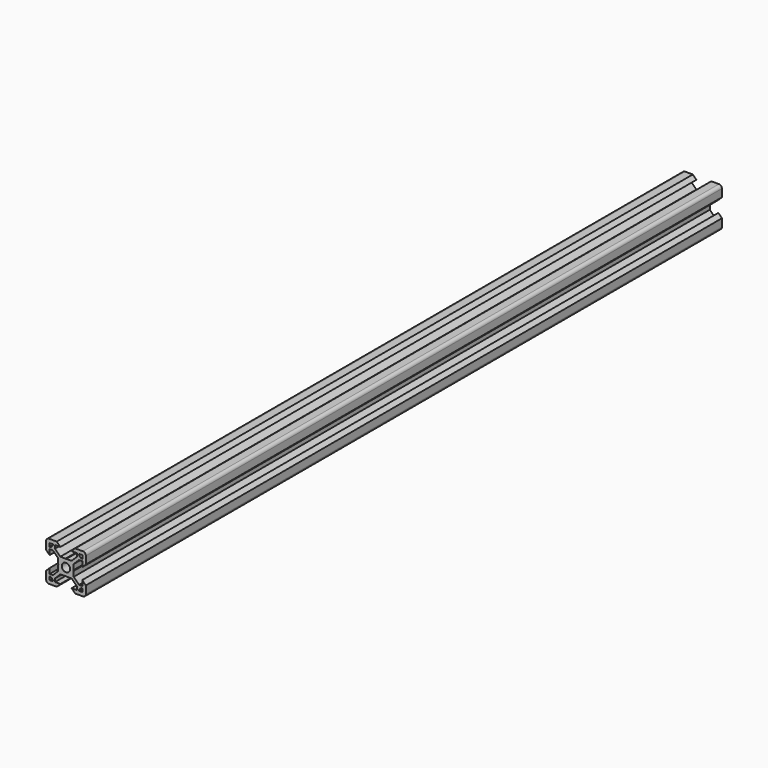
from build123d import *

# Parameters (mm, degrees)
F0_R     = 2.09999979
F1_DEPTH = 400


# Not quite as in the source:
# - ends of sketch curves that miss each other by under 0.0002 mm in the source are joined


with BuildPart() as f1:
    # F0 (on Front) → F1 (new body)
    with BuildSketch(Plane.XZ):
        with BuildLine():
            Line((-4.639999536, 10), (-8.50000015, 10))
            ThreePointArc((-8.50000015, 10), (-9.5606602157, 9.5606602157), (-10, 8.50000015))
            Line((-10, 8.50000015), (-10, 4.639999536))
            Line((-10, 4.639999536), (-8.19999818, 2.839999716))
            Line((-8.19999818, 2.839999716), (-8.19999818, 5.4993384501))
            Line((-8.19999818, 5.4993384501), (-6.559999344, 5.4993384501))
            Line((-6.559999344, 5.4993384501), (-3.9006596099, 2.839999716))
            Line((-3.9006596099, 2.839999716), (-3.9006596099, 0.19999898))
            Line((-3.9006596099, 0.19999898), (-3.7006596299, -1e-06))
            Line((-3.7006596299, -1e-06), (-3.9006596099, -0.20000098))
            Line((-3.9006596099, -0.20000098), (-3.9006596099, -2.840000716))
            Line((-3.9006596099, -2.840000716), (-6.559999344, -5.4993404501))
            Line((-6.559999344, -5.4993404501), (-8.19999818, -5.4993404501))
            Line((-8.19999818, -5.4993404501), (-8.19999818, -2.840000716))
            Line((-8.19999818, -2.840000716), (-10, -4.640000536))
            Line((-10, -4.640000536), (-10, -8.50000115))
            ThreePointArc((-10, -8.50000115), (-9.5606602157, -9.5606612157), (-8.50000015, -10.000001))
            Line((-8.50000015, -10.000001), (-4.639999536, -10))
            Line((-4.639999536, -10), (-2.839999716, -8.20000018))
            Line((-2.839999716, -8.20000018), (-5.4993394501, -8.20000018))
            Line((-5.4993394501, -8.20000018), (-5.4993394501, -6.560000344))
            Line((-5.4993394501, -6.560000344), (-2.839999716, -3.9006606099))
            Line((-2.839999716, -3.9006606099), (-0.19999898, -3.9006606099))
            Line((-0.19999898, -3.9006606099), (1e-06, -3.7006606299))
            Line((1e-06, -3.7006606299), (0.20000098, -3.9006606099))
            Line((0.20000098, -3.9006606099), (2.839999716, -3.9006606099))
            Line((2.839999716, -3.9006606099), (5.4993414501, -6.560000344))
            Line((5.4993414501, -6.560000344), (5.4993414501, -8.20000018))
            Line((5.4993414501, -8.20000018), (2.839999716, -8.20000018))
            Line((2.839999716, -8.20000018), (4.639999536, -10))
            Line((4.639999536, -10), (8.50000015, -10))
            ThreePointArc((8.50000015, -10), (9.5606602157, -9.5606612157), (10, -8.50000115))
            Line((10, -8.50000115), (10, -4.640000536))
            Line((10, -4.640000536), (8.20000018, -2.840000716))
            Line((8.20000018, -2.840000716), (8.20000018, -5.4993404501))
            Line((8.20000018, -5.4993404501), (6.560000344, -5.4993404501))
            Line((6.560000344, -5.4993404501), (3.9006596099, -2.840000716))
            Line((3.9006596099, -2.840000716), (3.9006596099, -0.20000098))
            Line((3.9006596099, -0.20000098), (3.7006596299, -1e-06))
            Line((3.7006596299, -1e-06), (3.9006596099, 0.19999898))
            Line((3.9006596099, 0.19999898), (3.9006596099, 2.839999716))
            Line((3.9006596099, 2.839999716), (6.560000344, 5.4993384501))
            Line((6.560000344, 5.4993384501), (8.20000018, 5.4993384501))
            Line((8.20000018, 5.4993384501), (8.20000018, 2.839999716))
            Line((8.20000018, 2.839999716), (10, 4.639999536))
            Line((10, 4.639999536), (10, 8.50000015))
            ThreePointArc((10, 8.50000015), (9.5606602157, 9.5606602157), (8.50000015, 10))
            Line((8.50000015, 10), (4.639999536, 10))
            Line((4.639999536, 10), (2.839999716, 8.20000018))
            Line((2.839999716, 8.20000018), (5.4993414501, 8.20000018))
            Line((5.4993414501, 8.20000018), (5.4993414501, 6.559998344))
            Line((5.4993414501, 6.559998344), (2.839999716, 3.9006596099))
            Line((2.839999716, 3.9006596099), (0.20000098, 3.9006596099))
            Line((0.20000098, 3.9006596099), (1e-06, 3.7006596299))
            Line((1e-06, 3.7006596299), (-0.19999898, 3.9006596099))
            Line((-0.19999898, 3.9006596099), (-2.839999716, 3.9006596099))
            Line((-2.839999716, 3.9006596099), (-5.4993394501, 6.559998344))
            Line((-5.4993394501, 6.559998344), (-5.4993394501, 8.20000018))
            Line((-5.4993394501, 8.20000018), (-2.839999716, 8.20000018))
            Line((-2.839999716, 8.20000018), (-4.639999536, 10))
        make_face()
        Polygon((-6.5693393431, -8.20000018), (-8.19999818, -8.20000018), (-8.19999818, -6.5693403431), (-7.629998237, -6.5693403431), (-6.5693393431, -7.630000237), align=None, mode=Mode.SUBTRACT)
        Polygon((8.20000018, -8.20000018), (6.5693393431, -8.20000018), (6.5693393431, -7.630000237), (7.630002237, -6.5693403431), (8.20000018, -6.5693403431), align=None, mode=Mode.SUBTRACT)
        with Locations((1e-06, -1e-06)):
            Circle(F0_R, mode=Mode.SUBTRACT)
        Polygon((-8.19999818, 8.20000018), (-6.5693393431, 8.20000018), (-6.5693393431, 7.629999237), (-7.629998237, 6.5693393431), (-8.19999818, 6.5693393431), align=None, mode=Mode.SUBTRACT)
        Polygon((6.5693393431, 8.20000018), (8.20000018, 8.20000018), (8.20000018, 6.5693393431), (7.630002237, 6.5693393431), (6.5693393431, 7.629999237), align=None, mode=Mode.SUBTRACT)
    extrude(amount=F1_DEPTH)


solid = f1.part
